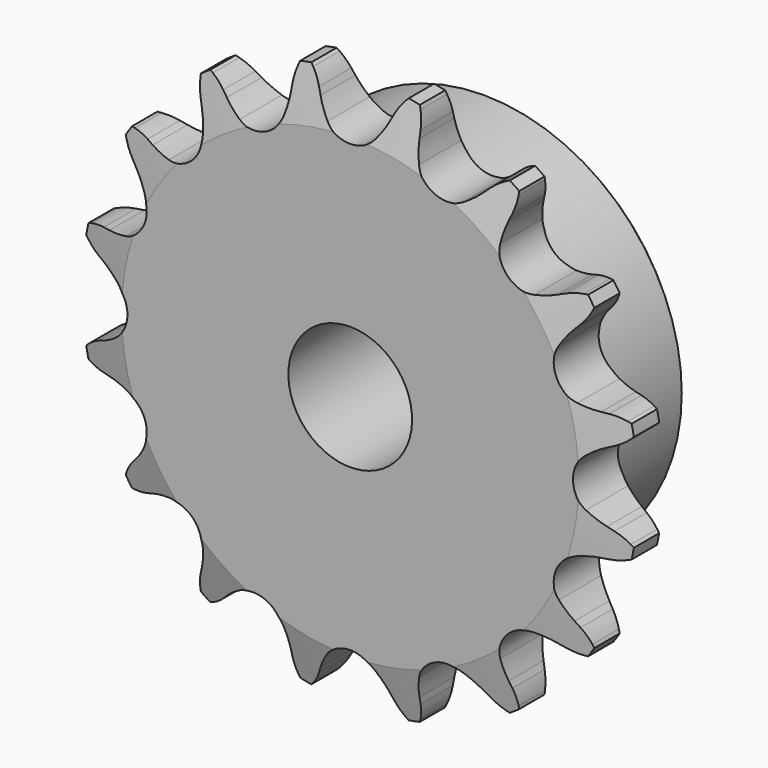
from build123d import *

# Parameters (mm, degrees)
F0_W         = 7.2136
F0_H         = 17.4625
F0_W_2       = 15.0114
F0_H_2       = 10.287
F3_R         = 1.5875
F4_SIZE      = 0.79375
F5_SIZE2     = 6.35
F5_SIZE      = 1.5748
F6_DEPTH     = 25.4
F7_TEXT_SIZE = 3.4981575381
F8_DEPTH     = 3.175


# Not quite as in the source:
# - ends of sketch curves that miss each other by under 0.0002 mm in the source are joined
# - Text() gives the source's letters only with a copy of the font that has no kerning and outlines rounded to 1/6400 em; it was checked with that copy


with BuildPart() as f1:
    # F0 (on Right) → F1 (revolve)
    with BuildSketch(Plane.YZ):
        with Locations((3.6068, 16.66875)):
            Rectangle(F0_W, F0_H)
        with Locations((14.7193, 16.66875)):
            Rectangle(F0_W_2, F0_H)
        with Locations((3.6068, 30.5435)):
            Rectangle(F0_W, F0_H_2)
    revolve(axis=Axis((0, 11.1125, 0), (0, 1, 0)))

    # F3
    f3_edges = [f1.edges().sort_by_distance(p)[0] for p in [
        (0, 7.2136, -25.4),
    ]]
    fillet(f3_edges, radius=F3_R)

    # F4
    f4_edges = [f1.edges().sort_by_distance(p)[0] for p in [
        (0, 22.225, -25.4),
    ]]
    chamfer(f4_edges, length=F4_SIZE)

    # F5
    f5_edges = [f1.edges().sort_by_distance(p)[0] for p in [
        (0, 0, -35.687),
        (0, 7.2136, -35.687),
    ]]
    f5_side = f1.faces().sort_by_distance((0, 3.6068, -35.687))[0]
    chamfer(f5_edges, length=F5_SIZE, length2=F5_SIZE2, reference=f5_side)

    # F2 (on face) → F6 (intersect)
    with BuildSketch(Plane.XZ):
        with BuildLine():
            ThreePointArc((-3.0901927561, 30.0699209737), (-3.8441744321, 31.1417339748), (-4.4568662909, 32.3001294872))
            Line((-4.4568662909, 32.3001294872), (-4.8163939581, 33.0982513131))
            ThreePointArc((-4.8163939581, 33.0982513131), (-5.3095043503, 33.998365289), (-5.9363686156, 34.8110178725))
            ThreePointArc((-5.9363686156, 34.8110178725), (-6.5023240211, 35.3660448432), (-7.1308152658, 35.8491175235))
            ThreePointArc((-7.1308152658, 35.8491175235), (-7.5265954308, 35.1623131557), (-7.8370704233, 34.4329533418))
            ThreePointArc((-7.8370704233, 34.4329533418), (-8.1052288122, 33.4422696854), (-8.2163447096, 32.4219676292))
            Line((-8.2163447096, 32.4219676292), (-8.2430769669, 31.5470139282))
            ThreePointArc((-8.2430769669, 31.5470139282), (-8.3658316701, 30.2423290008), (-8.6522548362, 28.963566612))
            ThreePointArc((-8.6522548362, 28.963566612), (-10.9400115583, 26.4115808479), (-14.3622262878, 26.5984190262))
            ThreePointArc((-14.3622262878, 26.5984190262), (-15.4689796012, 27.3001088298), (-16.4783318362, 28.1358597154))
            Line((-16.4783318362, 28.1358597154), (-17.1159200863, 28.7356428559))
            ThreePointArc((-17.1159200863, 28.7356428559), (-17.9159533879, 29.3785345614), (-18.8060891299, 29.8894370856))
            ThreePointArc((-18.8060891299, 29.8894370856), (-19.5413633702, 30.1856333901), (-20.306877478, 30.3914211689))
            ThreePointArc((-20.306877478, 30.3914211689), (-20.4097021653, 29.6054380607), (-20.4174297389, 28.8127838209))
            ThreePointArc((-20.4174297389, 28.8127838209), (-20.2860575636, 27.794891695), (-19.9982625737, 26.8097332954))
            Line((-19.9982625737, 26.8097332954), (-19.6881296734, 25.9911514873))
            ThreePointArc((-19.6881296734, 25.9911514873), (-19.3022589246, 24.7388035954), (-19.0775182449, 23.4477717972))
            ThreePointArc((-19.0775182449, 23.4477717972), (-20.2145271833, 20.2145577873), (-23.4477412028, 19.0775488761))
            ThreePointArc((-23.4477412028, 19.0775488761), (-24.7387729991, 19.3022895668), (-25.9911208877, 19.6881603261))
            Line((-25.9911208877, 19.6881603261), (-26.8097026932, 19.9982932333))
            ThreePointArc((-26.8097026932, 19.9982932333), (-27.7948610904, 20.2860882315), (-28.8127532152, 20.4174604154))
            ThreePointArc((-28.8127532152, 20.4174604154), (-29.6054074551, 20.4097328485), (-30.3914018446, 20.3069063988))
            ThreePointArc((-30.3914018446, 20.3069063988), (-30.1856167548, 19.5414033881), (-29.8894204565, 18.8061291453))
            ThreePointArc((-29.8894204565, 18.8061291453), (-29.3785179398, 17.9159933989), (-28.7356262411, 17.115960092))
            Line((-28.7356262411, 17.115960092), (-28.1358431059, 16.4783718368))
            ThreePointArc((-28.1358431059, 16.4783718368), (-27.3000922288, 15.4690195947), (-26.5984024345, 14.3622662754))
            ThreePointArc((-26.5984024345, 14.3622662754), (-26.4115642851, 10.9400515443), (-28.9635500685, 8.6522948437))
            ThreePointArc((-28.9635500685, 8.6522948437), (-30.2423124597, 8.3658716884), (-31.5469973882, 8.2431169963))
            Line((-31.5469973882, 8.2431169963), (-32.4219510894, 8.2163847464))
            ThreePointArc((-32.4219510894, 8.2163847464), (-33.4422531466, 8.1052688576), (-34.4329368052, 7.837110477))
            ThreePointArc((-34.4329368052, 7.837110477), (-35.1622966218, 7.5266354907), (-35.8491107721, 7.1308492074))
            ThreePointArc((-35.8491107721, 7.1308492074), (-35.3660448197, 6.5023671883), (-34.811017851, 5.9364117809))
            ThreePointArc((-34.811017851, 5.9364117809), (-33.9983652698, 5.3095475126), (-33.0982512957, 4.8164371172))
            Line((-33.0982512957, 4.8164371172), (-32.3001294711, 4.4569094471))
            ThreePointArc((-32.3001294711, 4.4569094471), (-31.1417339609, 3.8442175841), (-30.0699209625, 3.0902359042))
            ThreePointArc((-30.0699209625, 3.0902359042), (-28.5876801399, 2.16231e-05), (-30.0699209849, -3.0901926474))
            ThreePointArc((-30.0699209849, -3.0901926474), (-31.1417339887, -3.8441743196), (-32.3001295033, -4.4568661741))
            Line((-32.3001295033, -4.4568661741), (-33.0982513305, -4.8163938385))
            ThreePointArc((-33.0982513305, -4.8163938385), (-33.9983653082, -5.3095042274), (-34.8110178939, -5.9363684898))
            ThreePointArc((-34.8110178939, -5.9363684898), (-35.3660448667, -6.5023238932), (-35.8491175493, -7.1308151362))
            ThreePointArc((-35.8491175493, -7.1308151362), (-35.1623131467, -7.5265954732), (-34.4329533323, -7.8370704648))
            ThreePointArc((-34.4329533323, -7.8370704648), (-33.4422696756, -8.1052288525), (-32.4219676193, -8.2163447487))
            Line((-32.4219676193, -8.2163447487), (-31.5470139183, -8.2430770049))
            ThreePointArc((-31.5470139183, -8.2430770049), (-30.2423289907, -8.3658317065), (-28.9635666015, -8.6522548711))
            ThreePointArc((-28.9635666015, -8.6522548711), (-26.4115808347, -10.9400115901), (-26.5984190088, -14.3622263199))
            ThreePointArc((-26.5984190088, -14.3622263199), (-27.3001088112, -15.4689796341), (-28.1358596955, -16.4783318701))
            Line((-28.1358596955, -16.4783318701), (-28.7356428353, -17.115920121))
            ThreePointArc((-28.7356428353, -17.115920121), (-29.3785345398, -17.9159534233), (-29.889437063, -18.8060891659))
            ThreePointArc((-29.889437063, -18.8060891659), (-30.1856333665, -19.5413634066), (-30.3914211444, -20.3068775146))
            ThreePointArc((-30.3914211444, -20.3068775146), (-29.6054380361, -20.4097022009), (-28.8127837963, -20.4174297736))
            ThreePointArc((-28.8127837963, -20.4174297736), (-27.7948916705, -20.2860575971), (-26.8097332713, -19.998262606))
            Line((-26.8097332713, -19.998262606), (-25.9911514635, -19.6881297047))
            ThreePointArc((-25.9911514635, -19.6881297047), (-24.7388035721, -19.3022589544), (-23.4477717742, -19.0775182731))
            ThreePointArc((-23.4477717742, -19.0775182731), (-20.2145577629, -20.2145272077), (-19.0775488479, -23.4477412258))
            ThreePointArc((-19.0775488479, -23.4477412258), (-19.302289537, -24.7387730223), (-19.6881602948, -25.9911209114))
            Line((-19.6881602948, -25.9911209114), (-19.998293201, -26.8097027173))
            ThreePointArc((-19.998293201, -26.8097027173), (-20.286088198, -27.7948611148), (-20.4174603807, -28.8127532399))
            ThreePointArc((-20.4174603807, -28.8127532399), (-20.4097328128, -29.6054074796), (-20.3069063622, -30.3914018691))
            ThreePointArc((-20.3069063622, -30.3914018691), (-19.5414033517, -30.1856167783), (-18.8061291093, -29.8894204792))
            ThreePointArc((-18.8061291093, -29.8894204792), (-17.9159933635, -29.3785179614), (-17.1159600573, -28.7356262617))
            Line((-17.1159600573, -28.7356262617), (-16.4783718028, -28.1358431258))
            ThreePointArc((-16.4783718028, -28.1358431258), (-15.4690195618, -27.3000922475), (-14.3622662434, -26.5984024518))
            ThreePointArc((-14.3622662434, -26.5984024518), (-10.9400515125, -26.4115642983), (-8.6522948088, -28.9635500789))
            ThreePointArc((-8.6522948088, -28.9635500789), (-8.365871652, -30.2423124698), (-8.2431169582, -31.5469973982))
            Line((-8.2431169582, -31.5469973982), (-8.2163847073, -32.4219510993))
            ThreePointArc((-8.2163847073, -32.4219510993), (-8.1052688173, -33.4422531563), (-7.8371104355, -34.4329368146))
            ThreePointArc((-7.8371104355, -34.4329368146), (-7.5266354483, -35.1622966308), (-7.1308491642, -35.8491107807))
            ThreePointArc((-7.1308491642, -35.8491107807), (-6.5023671457, -35.3660448275), (-5.936411739, -34.8110178582))
            ThreePointArc((-5.936411739, -34.8110178582), (-5.3095474717, -33.9983652762), (-4.8164370773, -33.0982513015))
            Line((-4.8164370773, -33.0982513015), (-4.4569094082, -32.3001294765))
            ThreePointArc((-4.4569094082, -32.3001294765), (-3.8442175466, -31.1417339655), (-3.090235868, -30.0699209662))
            ThreePointArc((-3.090235868, -30.0699209662), (-2.15886e-05, -28.5876801399), (3.0901926836, -30.0699209811))
            ThreePointArc((3.0901926836, -30.0699209811), (3.8441743571, -31.141733984), (4.4568662131, -32.300129498))
            Line((4.4568662131, -32.300129498), (4.8163938783, -33.0982513247))
            ThreePointArc((4.8163938783, -33.0982513247), (5.3095042684, -33.9983653018), (5.9363685317, -34.8110178868))
            ThreePointArc((5.9363685317, -34.8110178868), (6.5023239358, -35.3660448589), (7.1308151794, -35.8491175407))
            ThreePointArc((7.1308151794, -35.8491175407), (7.5265955156, -35.1623131376), (7.8370705063, -34.4329533229))
            ThreePointArc((7.8370705063, -34.4329533229), (8.1052288928, -33.4422696659), (8.2163447878, -32.4219676094))
            Line((8.2163447878, -32.4219676094), (8.2430770429, -31.5470139084))
            ThreePointArc((8.2430770429, -31.5470139084), (8.365831743, -30.2423289806), (8.652254906, -28.9635665911))
            ThreePointArc((8.652254906, -28.9635665911), (10.940011622, -26.4115808215), (14.3622263519, -26.5984189915))
            ThreePointArc((14.3622263519, -26.5984189915), (15.468979667, -27.3001087925), (16.478331904, -28.1358596757))
            Line((16.478331904, -28.1358596757), (17.1159201556, -28.7356428147))
            ThreePointArc((17.1159201556, -28.7356428147), (17.9159534587, -29.3785345182), (18.806089202, -29.8894370403))
            ThreePointArc((18.806089202, -29.8894370403), (19.5413634429, -30.185633343), (20.3068775513, -30.3914211199))
            ThreePointArc((20.3068775513, -30.3914211199), (20.4097022366, -29.6054380115), (20.4174298083, -28.8127837717))
            ThreePointArc((20.4174298083, -28.8127837717), (20.2860576306, -27.7948916461), (19.9982626383, -26.8097332472))
            Line((19.9982626383, -26.8097332472), (19.688129736, -25.9911514398))
            ThreePointArc((19.688129736, -25.9911514398), (19.3022589842, -24.7388035489), (19.0775183014, -23.4477717512))
            ThreePointArc((19.0775183014, -23.4477717512), (20.214527232, -20.2145577386), (23.4477412488, -19.0775488196))
            ThreePointArc((23.4477412488, -19.0775488196), (24.7387730456, -19.3022895071), (25.9911209352, -19.6881602635))
            Line((25.9911209352, -19.6881602635), (26.8097027414, -19.9982931687))
            ThreePointArc((26.8097027414, -19.9982931687), (27.7948611393, -20.2860881645), (28.8127532645, -20.417460346))
            ThreePointArc((28.8127532645, -20.417460346), (29.6054075042, -20.4097327771), (30.3914018936, -20.3069063255))
            ThreePointArc((30.3914018936, -20.3069063255), (30.1856168019, -19.5414033153), (29.8894205018, -18.8061290732))
            ThreePointArc((29.8894205018, -18.8061290732), (29.378517983, -17.9159933281), (28.7356262823, -17.1159600227))
            Line((28.7356262823, -17.1159600227), (28.1358431456, -16.4783717689))
            ThreePointArc((28.1358431456, -16.4783717689), (27.3000922661, -15.4690195289), (26.5984024691, -14.3622662113))
            ThreePointArc((26.5984024691, -14.3622662113), (26.4115643115, -10.9400514807), (28.9635500894, -8.6522947739))
            ThreePointArc((28.9635500894, -8.6522947739), (30.2423124799, -8.3658716156), (31.5469974081, -8.2431169202))
            Line((31.5469974081, -8.2431169202), (32.4219511092, -8.2163846682))
            ThreePointArc((32.4219511092, -8.2163846682), (33.4422531661, -8.105268777), (34.4329368241, -7.837110394))
            ThreePointArc((34.4329368241, -7.837110394), (35.1622966399, -7.5266354059), (35.8491107893, -7.130849121))
            ThreePointArc((35.8491107893, -7.130849121), (35.3660448354, -6.5023671031), (34.8110178653, -5.936411697))
            ThreePointArc((34.8110178653, -5.936411697), (33.9983652826, -5.3095474307), (33.0982513073, -4.8164370374))
            Line((33.0982513073, -4.8164370374), (32.3001294819, -4.4569093693))
            ThreePointArc((32.3001294819, -4.4569093693), (31.1417339701, -3.8442175091), (30.06992097, -3.0902358318))
            ThreePointArc((30.06992097, -3.0902358318), (28.5876801399, -2.15542e-05), (30.0699209774, 3.0901927199))
            ThreePointArc((30.0699209774, 3.0901927199), (31.1417339794, 3.8441743946), (32.3001294926, 4.456866252))
            Line((32.3001294926, 4.456866252), (33.0982513189, 4.8163939182))
            ThreePointArc((33.0982513189, 4.8163939182), (33.9983652954, 5.3095043093), (34.8110178796, 5.9363685737))
            ThreePointArc((34.8110178796, 5.9363685737), (35.366044851, 6.5023239784), (35.8491175321, 7.1308152226))
            ThreePointArc((35.8491175321, 7.1308152226), (35.1623131285, 7.5265955579), (34.4329533134, 7.8370705478))
            ThreePointArc((34.4329533134, 7.8370705478), (33.4422696561, 8.1052289331), (32.4219675995, 8.2163448268))
            Line((32.4219675995, 8.2163448268), (31.5470138984, 8.2430770809))
            ThreePointArc((31.5470138984, 8.2430770809), (30.2423289705, 8.3658317794), (28.9635665807, 8.6522549409))
            ThreePointArc((28.9635665807, 8.6522549409), (26.4115808083, 10.9400116538), (26.5984189742, 14.362226384))
            ThreePointArc((26.5984189742, 14.362226384), (27.3001087739, 15.4689796998), (28.1358596558, 16.4783319379))
            Line((28.1358596558, 16.4783319379), (28.735642794, 17.1159201902))
            ThreePointArc((28.735642794, 17.1159201902), (29.3785344966, 17.9159534941), (29.8894370176, 18.806089238))
            ThreePointArc((29.8894370176, 18.806089238), (30.1856333194, 19.5413634793), (30.3914210955, 20.3068775879))
            ThreePointArc((30.3914210955, 20.3068775879), (29.6054379869, 20.4097022723), (28.8127837471, 20.4174298431))
            ThreePointArc((28.8127837471, 20.4174298431), (27.7948916217, 20.2860576641), (26.8097332231, 19.9982626706))
            Line((26.8097332231, 19.9982626706), (25.9911514161, 19.6881297674))
            ThreePointArc((25.9911514161, 19.6881297674), (24.7388035256, 19.3022590141), (23.4477717282, 19.0775183296))
            ThreePointArc((23.4477717282, 19.0775183296), (20.2145577142, 20.2145272564), (19.0775487914, 23.4477412718))
            ThreePointArc((19.0775487914, 23.4477412718), (19.3022894773, 24.7387730689), (19.6881602321, 25.9911209589))
            Line((19.6881602321, 25.9911209589), (19.9982931364, 26.8097027655))
            ThreePointArc((19.9982931364, 26.8097027655), (20.286088131, 27.7948611637), (20.4174603112, 28.8127532891))
            ThreePointArc((20.4174603112, 28.8127532891), (20.4097327414, 29.6054075288), (20.3069062889, 30.391401918))
            ThreePointArc((20.3069062889, 30.391401918), (19.5414032789, 30.1856168254), (18.8061290372, 29.8894205245))
            ThreePointArc((18.8061290372, 29.8894205245), (17.9159932927, 29.3785180046), (17.1159599881, 28.7356263029))
            Line((17.1159599881, 28.7356263029), (16.478371735, 28.1358431655))
            ThreePointArc((16.478371735, 28.1358431655), (15.469019496, 27.3000922848), (14.3622661793, 26.5984024865))
            ThreePointArc((14.3622661793, 26.5984024865), (10.9400514489, 26.4115643247), (8.652294739, 28.9635500998))
            ThreePointArc((8.652294739, 28.9635500998), (8.3658715791, 30.24231249), (8.2431168822, 31.546997418))
            Line((8.2431168822, 31.546997418), (8.2163846291, 32.4219511191))
            ThreePointArc((8.2163846291, 32.4219511191), (8.1052687366, 33.4422531759), (7.8371103525, 34.4329368335))
            ThreePointArc((7.8371103525, 34.4329368335), (7.5266353635, 35.162296649), (7.1308490778, 35.8491107979))
            ThreePointArc((7.1308490778, 35.8491107979), (6.5023670605, 35.3660448432), (5.9364116551, 34.8110178725))
            ThreePointArc((5.9364116551, 34.8110178725), (5.3095473897, 33.998365289), (4.8164369975, 33.0982513131))
            Line((4.8164369975, 33.0982513131), (4.4569093303, 32.3001294872))
            ThreePointArc((4.4569093303, 32.3001294872), (3.8442174716, 31.1417339748), (3.0902357955, 30.0699209737))
            ThreePointArc((3.0902357955, 30.0699209737), (2.15197e-05, 28.5876801399), (-3.0901927561, 30.0699209737))
        make_face()
    extrude(amount=-F6_DEPTH, mode=Mode.INTERSECT)

    # F7 (on face) → F8 (cut)
    with BuildSketch(Plane(origin=(0, 22.225, 0), x_dir=(-1, 0, 0), z_dir=(0, 1, 0))):
        with Locations((-14.4133095164, -11.9767310098)):
            Text('Designed on iPad', F7_TEXT_SIZE, font='Open Sans', font_style=FontStyle.BOLD, text_align=(TextAlign.LEFT, TextAlign.BOTTOM))
        with Locations((-12.5953607708, -16.7342252615)):
            Text('using OnShape', F7_TEXT_SIZE, font='Open Sans', font_style=FontStyle.BOLD, text_align=(TextAlign.LEFT, TextAlign.BOTTOM))
    extrude(amount=-F8_DEPTH, mode=Mode.SUBTRACT)


solid = f1.part
